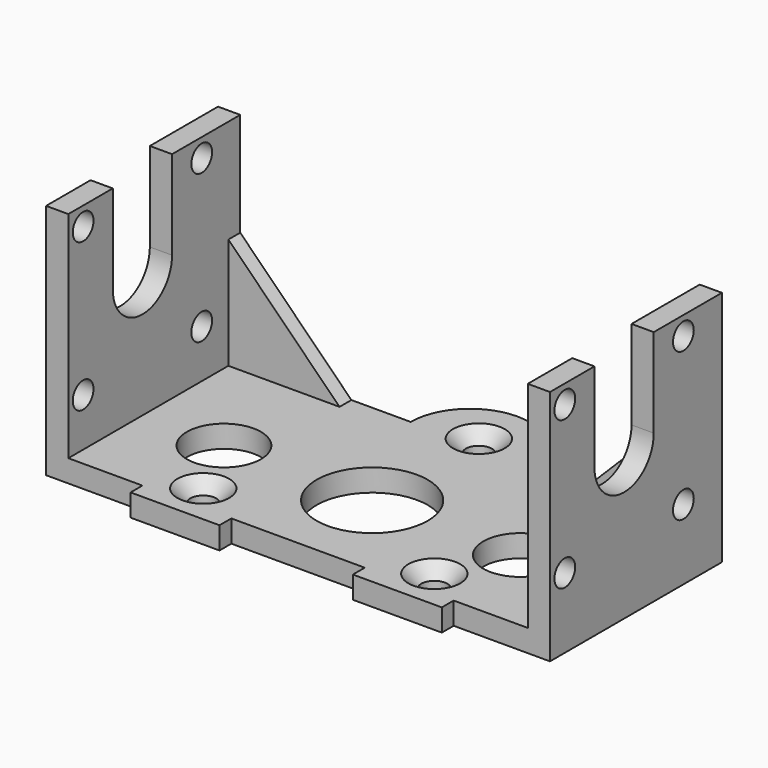
from build123d import *

# Parameters (mm, degrees)
F0_W            = 12
F0_H            = 2
F1_DEPTH        = 3
F2_W            = 3
F2_H            = 29
F3_DEPTH        = 29
F4_W            = 15
F4_H            = 2
F5_DEPTH        = 15
F6_SIZE         = 14.99999
F8_D            = 3.5
F10_D           = 3.5
F10_CSINK_D     = 7
F10_CSINK_ANGLE = 90
F11_R           = 7.5
F11_R_2         = 5
F12_DEPTH       = 25
F13_W           = 10
F13_H           = 12
F14_DEPTH       = 68.001


# Not quite as in the source:
# - a fillet or chamfer is up to 0.001 mm smaller than in the source, because OpenCascade refuses the exact size
# - a feature names something its author has since deleted; it is built from what else it names


with BuildPart() as f1:
    # F0 (on Top) → F1 (new body)
    with BuildSketch(Plane.XY):
        Polygon((34, -12.5), (34, 16.5), (8, 16.5), (-8, 16.5), (-34, 16.5), (-34, -12.5), (-21, -12.5), (-9, -12.5), (9, -12.5), (21, -12.5), align=None)
        with BuildLine():
            Line((-8, 16.5), (8, 16.5))
            ThreePointArc((8, 16.5), (0, 24.5), (-8, 16.5))
        make_face()
        with Locations((-15, -13.5)):
            Rectangle(F0_W, F0_H)
        with Locations((15, -13.5)):
            Rectangle(F0_W, F0_H)
    extrude(amount=F1_DEPTH)

    # F2 (on face) → F3 (join)
    with BuildSketch(Plane.XY.offset(3)):
        with Locations((-32.5, 2)):
            Rectangle(F2_W, F2_H)
        with Locations((32.5, 2)):
            Rectangle(F2_W, F2_H)
    extrude(amount=F3_DEPTH)

    # F4 (on face) → F5 (join)
    with BuildSketch(Plane.XY.offset(3)):
        with Locations((-23.5, 15.5)):
            Rectangle(F4_W, F4_H)
        with Locations((23.5, 15.5)):
            Rectangle(F4_W, F4_H)
    extrude(amount=F5_DEPTH)

    # F6 (size 15 in the source; OpenCascade refuses exactly that, so slightly less here)
    f6_edges = [f1.edges().sort_by_distance(p)[0] for p in [
        (-16, 15.5, 18),
        (16, 15.5, 18),
    ]]
    chamfer(f6_edges, length=F6_SIZE)

    # F8 (through all)
    with Locations(Plane(origin=(-34, 0, 0), x_dir=(0, -1, 0), z_dir=(-1, 0, 0))):
        with Locations((10, 29.5), (10, 9.5), (-10, 9.5), (-10, 29.5)):
            Hole(F8_D / 2)

    # F10 (through all)
    with Locations(Plane.XY.offset(3)):
        with Locations((0, 18), (-15.5884572681, -9), (15.5884572681, -9)):
            CounterSinkHole(F10_D / 2, F10_CSINK_D / 2, counter_sink_angle=F10_CSINK_ANGLE)

    # F11 (on face) → F12 (cut)
    with BuildSketch(Plane(origin=(0, 0, 0), x_dir=(1, 0, 0), z_dir=(0, 0, -1))):
        Circle(F11_R)
        with Locations((20, 0)):
            Circle(F11_R_2)
        with Locations((-20, 0)):
            Circle(F11_R_2)
    extrude(amount=-F12_DEPTH, mode=Mode.SUBTRACT)

    # F13 (on face) → F14 (cut, through all)
    with BuildSketch(Plane.YZ.offset(34)):
        with Locations((0, 26)):
            Rectangle(F13_W, F13_H)
        with BuildLine():
            ThreePointArc((-5, 20), (0, 15), (5, 20))
            Line((5, 20), (-5, 20))
        make_face()
    extrude(amount=-F14_DEPTH, mode=Mode.SUBTRACT)


solid = f1.part
